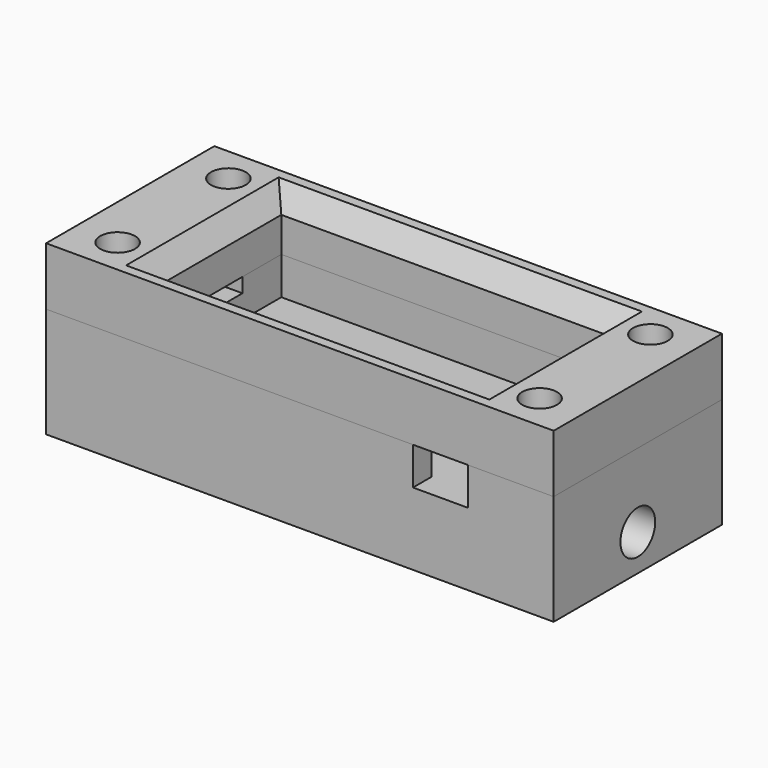
from build123d import *

# Parameters (mm, degrees)
F1_DEPTH       = 2.6
F2_W           = 3.55
F2_H           = 4.6
F3_DEPTH       = 1.6
F4_W           = 35
F4_H           = 14.5
F5_DEPTH       = 5
F6_R           = 1.5
F7_DEPTH       = 8.5
F8_W           = 35
F8_H           = 14.5
F8_W_2         = 23.2
F8_H_2         = 11.3
F9_DEPTH       = 4
F10_R          = 1.2
F11_DEPTH      = 5.5
F11_DEPTH_BACK = 4.001
F12_C1_SIZE2   = 1.6
F12_C1_SIZE    = 0.9237604307
F12_C2_SIZE2   = 1.6
F12_C2_SIZE    = 0.9237604307
F12_C3_SIZE2   = 1.6
F12_C3_SIZE    = 0.9237604307
F12_C4_SIZE2   = 1.6
F12_C4_SIZE    = 0.9237604307


# Not quite as in the source:
# - a pattern or mirror of a feature is missing from the dataset's text; its kind, count and spacing are read off the source's solid


with BuildPart() as f1:
    # F0 (on Top) → F1 (new body)
    with BuildSketch(Plane.XY):
        Polygon((17.5, -7.25), (17.5, 7.25), (-17.5, 7.25), (-17.5, -7.25), (7.8, -7.25), (7.8, -5.65), (-11.6, -5.65), (-11.6, -2.3), (-15.15, -2.3), (-15.15, 2.3), (-11.6, 2.3), (-11.6, 5.65), (11.6, 5.65), (11.6, 2.3), (15.15, 2.3), (15.15, -2.3), (11.6, -2.3), (11.6, -7.25), align=None)
    extrude(amount=-F1_DEPTH)

    # F2 (on face) → F3 (join, through all)
    with BuildSketch(Plane(origin=(0, 0, -2.6), x_dir=(1, 0, 0), z_dir=(0, 0, -1))):
        with Locations((-13.375, 0)):
            Rectangle(F2_W, F2_H)
        with Locations((13.375, 0)):
            Rectangle(F2_W, F2_H)
    extrude(amount=-F3_DEPTH)

    # F4 (on face) → F5 (join)
    with BuildSketch(Plane(origin=(0, 0, -2.6), x_dir=(1, 0, 0), z_dir=(0, 0, -1))):
        Rectangle(F4_W, F4_H)
    extrude(amount=F5_DEPTH)

    # F6 (on face) → F7 (cut)
    with BuildSketch(Plane(origin=(-17.5, 0, 0), x_dir=(0, -1, 0), z_dir=(-1, 0, 0))):
        with Locations((0, -5.1)):
            Circle(F6_R)
    f7 = extrude(amount=-F7_DEPTH, mode=Mode.SUBTRACT)

    # F7_copies: F7 across plane
    add(f7.mirror(Plane(origin=(0, 0, 0), x_dir=(0, 0, 1), z_dir=(1, 0, 0))), mode=Mode.SUBTRACT)


with BuildPart() as f9:
    # F8 (on face) → F9 (new body)
    with BuildSketch(Plane.XY):
        Rectangle(F8_W, F8_H)
        Rectangle(F8_W_2, F8_H_2, mode=Mode.SUBTRACT)
    extrude(amount=F9_DEPTH)


with BuildPart() as f11_tool:
    # F10 (on face) → F11 (new body, two sides)
    with BuildSketch(Plane.XY) as f11_sk:
        with Locations((-14.55, 4.775)):
            Circle(F10_R)
        with Locations((14.55, 4.775)):
            Circle(F10_R)
        with Locations((-14.55, -4.775)):
            Circle(F10_R)
        with Locations((14.55, -4.775)):
            Circle(F10_R)
    extrude(amount=-F11_DEPTH)
    extrude(f11_sk.sketch, amount=F11_DEPTH_BACK)


with BuildPart() as f1_1:
    add(f1.part)

    # F11: cut by f11_tool
    add(f11_tool.part, mode=Mode.SUBTRACT)


with BuildPart() as f9_1:
    add(f9.part)

    # F11: cut by f11_tool
    add(f11_tool.part, mode=Mode.SUBTRACT)

    # F12: chamfer of 1.6 x 0.9237604307 on 4 edges, made by hand

    # F12_c1
    f12_c1_edges = [f9_1.edges().sort_by_distance(p)[0] for p in [
        (-11.6, 0, 4),
    ]]
    f12_c1_side = f9_1.faces().sort_by_distance((-11.6184752086, 0, 4))[0]
    chamfer(f12_c1_edges, length=F12_C1_SIZE, length2=F12_C1_SIZE2, reference=f12_c1_side)

    # F12_c2
    f12_c2_edges = [f9_1.edges().sort_by_distance(p)[0] for p in [
        (0, -5.65, 4),
    ]]
    f12_c2_side = f9_1.faces().sort_by_distance((0, -5.6684752086, 4))[0]
    chamfer(f12_c2_edges, length=F12_C2_SIZE, length2=F12_C2_SIZE2, reference=f12_c2_side)

    # F12_c3
    f12_c3_edges = [f9_1.edges().sort_by_distance(p)[0] for p in [
        (0, 5.65, 4),
    ]]
    f12_c3_side = f9_1.faces().sort_by_distance((0, 5.6684752086, 4))[0]
    chamfer(f12_c3_edges, length=F12_C3_SIZE, length2=F12_C3_SIZE2, reference=f12_c3_side)

    # F12_c4
    f12_c4_edges = [f9_1.edges().sort_by_distance(p)[0] for p in [
        (11.6, 0, 4),
    ]]
    f12_c4_side = f9_1.faces().sort_by_distance((11.6184752086, 0, 4))[0]
    chamfer(f12_c4_edges, length=F12_C4_SIZE, length2=F12_C4_SIZE2, reference=f12_c4_side)


solid = Compound([f1_1.part, f9_1.part])
